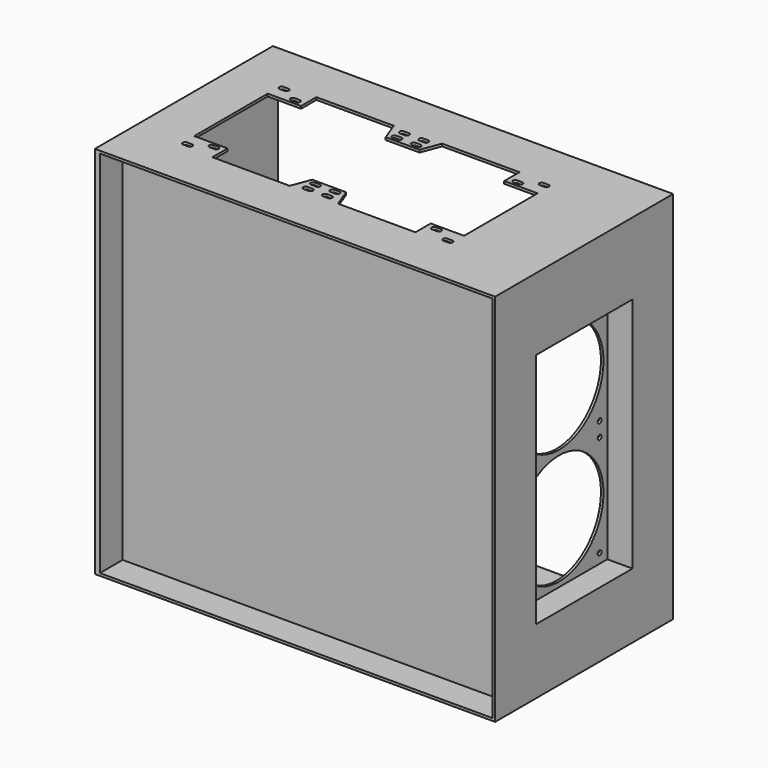
from build123d import *

# Parameters (mm, degrees)
F0_W      = 424
F0_H      = 397
F1_DEPTH  = 230
F2_W      = 406
F2_H      = 381.8
F3_DEPTH  = 230.001
F5_DEPTH  = 230.001
F6_W      = 10
F6_H      = 5
F7_DEPTH  = 2.6
F8_W      = 125
F8_H      = 245
F9_DEPTH  = 2.6
F10_W     = 130.2
F10_H     = 250.2
F10_W_2   = 125
F10_H_2   = 245
F11_DEPTH = 26
F12_W     = 125
F12_H     = 245
F13_DEPTH = 2.6
F14_R     = 2.5
F14_R_2   = 57.5
F15_DEPTH = 2.6
F16_R     = 2.49999
F20_W     = 406
F20_H     = 381.8
F21_DEPTH = 2.6


# Not quite as in the source:
# - a fillet or chamfer is up to 0.001 mm smaller than in the source, because OpenCascade refuses the exact size


with BuildPart() as f1:
    # F0 (on Front) → F1 (new body)
    with BuildSketch(Plane.XZ):
        with Locations((212, 198.5)):
            Rectangle(F0_W, F0_H)
    extrude(amount=F1_DEPTH)

    # F2 (on face) → F3 (cut, through all)
    with BuildSketch(Plane.XZ.offset(230)):
        with Locations((208.2, 193.5)):
            Rectangle(F2_W, F2_H)
    extrude(amount=-F3_DEPTH, mode=Mode.SUBTRACT)

    # F4 (on face) → F5 (cut, through all)
    with BuildSketch(Plane.XZ.offset(230)):
        Polygon((424, 397), (0, 397), (0, 387), (413.8, 387), (413.8, 0), (424, 0), align=None)
    extrude(amount=-F5_DEPTH, mode=Mode.SUBTRACT)

    # F6 (on face) → F7 (cut, through all)
    with BuildSketch(Plane.XY.offset(387)):
        Polygon((48.7, -67.5), (48.7, -115), (48.7, -162.5), (83.2, -162.5), (83.2, -182.25), (163.2, -182.25), (170.7, -162.5), (205.7, -162.5), (213.2, -182.25), (293.2, -182.25), (293.2, -162.5), (327.7, -162.5), (327.7, -115), (327.7, -67.5), (293.2, -67.5), (293.2, -47.75), (213.2, -47.75), (205.7, -67.5), (170.7, -67.5), (163.2, -47.75), (83.2, -47.75), (83.2, -67.5), align=None)
        with Locations((53.7, -52.75)):
            Rectangle(F6_W, F6_H)
        with Locations((73.2, -62.5)):
            Rectangle(F6_W, F6_H)
        with Locations((178.2, -52.75)):
            Rectangle(F6_W, F6_H)
        with Locations((178.2, -62.5)):
            Rectangle(F6_W, F6_H)
        with Locations((198.2, -52.75)):
            Rectangle(F6_W, F6_H)
        with Locations((198.2, -62.5)):
            Rectangle(F6_W, F6_H)
        with Locations((322.7, -52.75)):
            Rectangle(F6_W, F6_H)
        with Locations((303.2, -62.5)):
            Rectangle(F6_W, F6_H)
        with Locations((53.7, -177.25)):
            Rectangle(F6_W, F6_H)
        with Locations((73.2, -167.5)):
            Rectangle(F6_W, F6_H)
        with Locations((198.2, -177.25)):
            Rectangle(F6_W, F6_H)
        with Locations((178.2, -177.25)):
            Rectangle(F6_W, F6_H)
        with Locations((178.2, -167.5)):
            Rectangle(F6_W, F6_H)
        with Locations((198.2, -167.5)):
            Rectangle(F6_W, F6_H)
        with Locations((322.7, -177.25)):
            Rectangle(F6_W, F6_H)
        with Locations((303.2, -167.5)):
            Rectangle(F6_W, F6_H)
    extrude(amount=-F7_DEPTH, mode=Mode.SUBTRACT)

    # F8 (on face) → F9 (cut, through all)
    with BuildSketch(Plane.YZ.offset(413.8)):
        with Locations((-115, 189.9)):
            Rectangle(F8_W, F8_H)
    extrude(amount=-F9_DEPTH, mode=Mode.SUBTRACT)

    # F10 (on face) → F11 (join)
    with BuildSketch(Plane(origin=(411.2, 0, 0), x_dir=(0, -1, 0), z_dir=(-1, 0, 0))):
        with Locations((115, 189.9)):
            Rectangle(F10_W, F10_H)
        with Locations((115, 189.9)):
            Rectangle(F10_W_2, F10_H_2, mode=Mode.SUBTRACT)
    extrude(amount=F11_DEPTH)

    # F12 (on face) → F13 (join)
    with BuildSketch(Plane(origin=(385.2, 0, 0), x_dir=(0, -1, 0), z_dir=(-1, 0, 0))):
        with Locations((115, 189.9)):
            Rectangle(F12_W, F12_H)
    extrude(amount=-F13_DEPTH)

    # F14 (on face) → F15 (cut, through all)
    with BuildSketch(Plane.YZ.offset(387.8)):
        with Locations((-167.5, 302.4)):
            Circle(F14_R)
        with Locations((-62.5, 302.4)):
            Circle(F14_R)
        with Locations((-167.5, 197.4)):
            Circle(F14_R)
        with Locations((-62.5, 197.4)):
            Circle(F14_R)
        with Locations((-167.5, 182.4)):
            Circle(F14_R)
        with Locations((-62.5, 182.4)):
            Circle(F14_R)
        with Locations((-167.5, 77.4)):
            Circle(F14_R)
        with Locations((-62.5, 77.4)):
            Circle(F14_R)
        with Locations((-115, 249.9)):
            Circle(F14_R_2)
        with Locations((-115, 129.9)):
            Circle(F14_R_2)
    extrude(amount=-F15_DEPTH, mode=Mode.SUBTRACT)

    # F16 (radius 2.5 in the source; OpenCascade refuses exactly that, so slightly less here)
    f16_edges = [f1.edges().sort_by_distance(p)[0] for p in [
        (48.7, -50.25, 385.7),
        (58.7, -50.25, 385.7),
        (58.7, -55.25, 385.7),
        (48.7, -55.25, 385.7),
        (68.2, -60, 385.7),
        (68.2, -65, 385.7),
        (78.2, -65, 385.7),
        (78.2, -60, 385.7),
        (203.2, -65, 385.7),
        (193.2, -65, 385.7),
        (193.2, -60, 385.7),
        (203.2, -60, 385.7),
        (203.2, -55.25, 385.7),
        (193.2, -55.25, 385.7),
        (193.2, -50.25, 385.7),
        (203.2, -50.25, 385.7),
        (183.2, -50.25, 385.7),
        (173.2, -50.25, 385.7),
        (173.2, -55.25, 385.7),
        (183.2, -55.25, 385.7),
        (183.2, -60, 385.7),
        (173.2, -60, 385.7),
        (173.2, -65, 385.7),
        (183.2, -65, 385.7),
        (298.2, -60, 385.7),
        (298.2, -65, 385.7),
        (308.2, -65, 385.7),
        (308.2, -60, 385.7),
        (317.7, -55.25, 385.7),
        (317.7, -50.25, 385.7),
        (327.7, -50.25, 385.7),
        (327.7, -55.25, 385.7),
        (327.7, -174.75, 385.7),
        (327.7, -179.75, 385.7),
        (317.7, -179.75, 385.7),
        (317.7, -174.75, 385.7),
        (308.2, -170, 385.7),
        (308.2, -165, 385.7),
        (298.2, -165, 385.7),
        (298.2, -170, 385.7),
        (203.2, -165, 385.7),
        (193.2, -165, 385.7),
        (193.2, -170, 385.7),
        (203.2, -170, 385.7),
        (203.2, -174.75, 385.7),
        (193.2, -174.75, 385.7),
        (193.2, -179.75, 385.7),
        (203.2, -179.75, 385.7),
        (183.2, -179.75, 385.7),
        (183.2, -174.75, 385.7),
        (173.2, -174.75, 385.7),
        (173.2, -179.75, 385.7),
        (173.2, -165, 385.7),
        (173.2, -170, 385.7),
        (183.2, -170, 385.7),
        (183.2, -165, 385.7),
        (78.2, -165, 385.7),
        (78.2, -170, 385.7),
        (68.2, -170, 385.7),
        (68.2, -165, 385.7),
        (48.7, -174.75, 385.7),
        (48.7, -179.75, 385.7),
        (58.7, -179.75, 385.7),
        (58.7, -174.75, 385.7),
    ]]
    fillet(f16_edges, radius=F16_R)

    # F20 (on offset) → F21 (join)
    with BuildSketch(Plane.XZ.offset(198)):
        with Locations((208.2, 193.5)):
            Rectangle(F20_W, F20_H)
    extrude(amount=F21_DEPTH)


solid = f1.part
